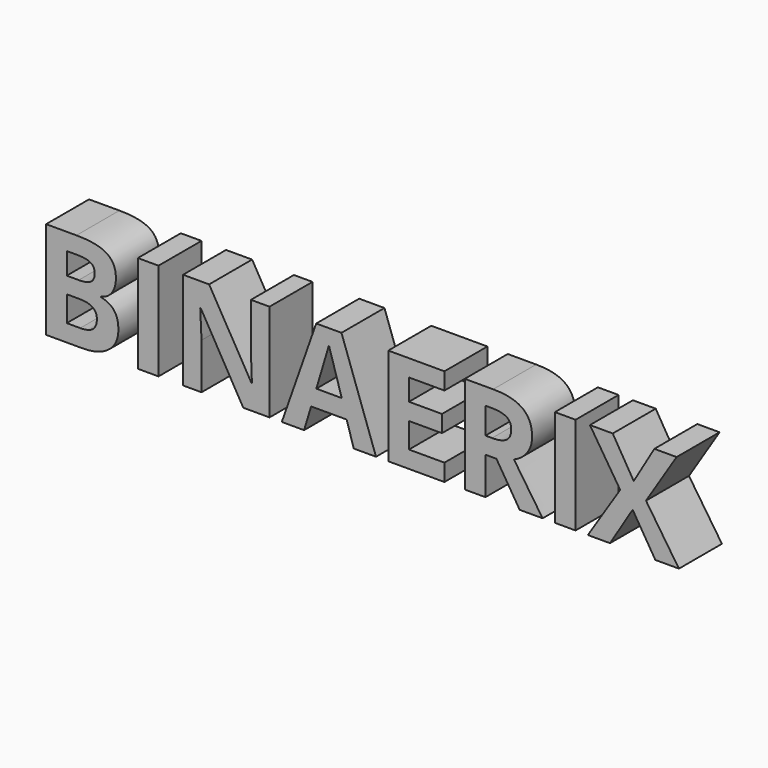
from build123d import *

# Parameters (mm, degrees)
F0_TEXT_SIZE = 32.2784323038
F1_DEPTH     = 12.7


# Not quite as in the source:
# - Text() gives the source's letters only with a copy of the font that has no kerning and outlines rounded to 1/6400 em; it was checked with that copy


with BuildPart() as f1:
    # F0 (on Front) → F1 (new body)
    with BuildSketch(Plane.XZ):
        with Locations((-80.8468163013, -14.9574056268)):
            Text('BINAERIX', F0_TEXT_SIZE, font='Open Sans', font_style=FontStyle.BOLD, text_align=(TextAlign.LEFT, TextAlign.BOTTOM))
    extrude(amount=F1_DEPTH)


solid = f1.part
